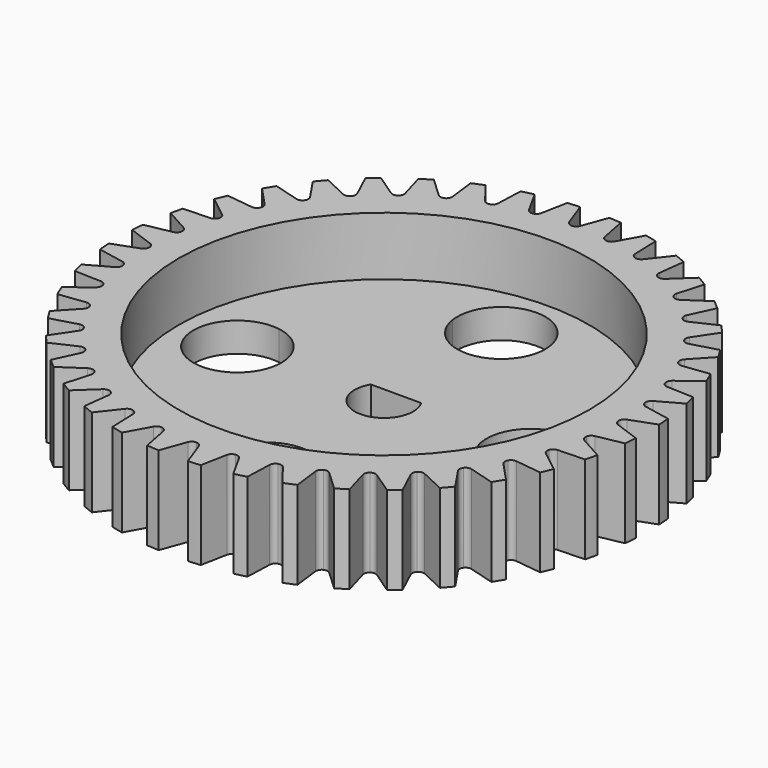
from build123d import *

# Parameters (mm, degrees)
F0_R            = 35
F0_R_2          = 10
F1_DEPTH        = 5
F2_DEPTH        = 15
F3_R            = 2
F4_DEPTH        = 32.4449635407
F0_R_3          = 45
F0_R_4          = 40
F5_DEPTH        = 5
F6_DEPTH        = 10
F8_DEPTH        = 25.0010001
F8_COPIES_COUNT = 40


# Not quite as in the source:
# - a feature of the source that left no trace in its solid (it failed there, or was rolled back) is left out
# - a pattern or mirror of a feature is missing from the dataset's text; its kind, count and spacing are read off the source's solid


with BuildPart() as f1:
    # F0 (on Top) → F1 (new body)
    with BuildSketch(Plane.XY):
        Circle(F0_R)
        with BuildLine():
            ThreePointArc((7.415144975, 23.875), (17.6776695297, 17.6776695297), (23.875, 7.415144975))
            ThreePointArc((23.875, 7.415144975), (29.8894018039, 5.687156583), (32.5, 0))
            ThreePointArc((32.5, 0), (29.8894018039, -5.687156583), (23.875, -7.415144975))
            ThreePointArc((23.875, -7.415144975), (17.6776695297, -17.6776695297), (7.415144975, -23.875))
            ThreePointArc((7.415144975, -23.875), (7.478756157, -24.4359021859), (7.5, -25))
            ThreePointArc((7.5, -25), (-0.5640978141, -32.478756157), (-7.415144975, -23.875))
            ThreePointArc((-7.415144975, -23.875), (-17.6776695297, -17.6776695297), (-23.875, -7.415144975))
            ThreePointArc((-23.875, -7.415144975), (-32.5, 0), (-23.875, 7.415144975))
            ThreePointArc((-23.875, 7.415144975), (-17.6776695297, 17.6776695297), (-7.415144975, 23.875))
            ThreePointArc((-7.415144975, 23.875), (-0.5640978141, 32.478756157), (7.5, 25))
            ThreePointArc((7.5, 25), (7.478756157, 24.4359021859), (7.415144975, 23.875))
        make_face(mode=Mode.SUBTRACT)
        with BuildLine():
            ThreePointArc((23.875, -7.415144975), (17.5, 0), (23.875, 7.415144975))
            ThreePointArc((23.875, 7.415144975), (17.6776695297, 17.6776695297), (7.415144975, 23.875))
            ThreePointArc((7.415144975, 23.875), (0, 17.5), (-7.415144975, 23.875))
            ThreePointArc((-7.415144975, 23.875), (-17.6776695297, 17.6776695297), (-23.875, 7.415144975))
            ThreePointArc((-23.875, 7.415144975), (-19.312843417, 4.8894018039), (-17.5, 0))
            ThreePointArc((-17.5, 0), (-19.312843417, -4.8894018039), (-23.875, -7.415144975))
            ThreePointArc((-23.875, -7.415144975), (-17.6776695297, -17.6776695297), (-7.415144975, -23.875))
            ThreePointArc((-7.415144975, -23.875), (0, -17.5), (7.415144975, -23.875))
            ThreePointArc((7.415144975, -23.875), (17.6776695297, -17.6776695297), (23.875, -7.415144975))
        make_face()
        Circle(F0_R_2, mode=Mode.SUBTRACT)
    extrude(amount=-F1_DEPTH)

    # F0 (on Top) → F2 (join)
    with BuildSketch(Plane.XY):
        Circle(F0_R_2)
        with BuildLine():
            ThreePointArc((5, 0), (-1.3254364946, -4.8211220788), (-4.2972872395, 2.5560364593))
            ThreePointArc((-4.2972872395, 2.5560364593), (0, 5), (4.2972872395, 2.5560364593))
            ThreePointArc((4.2972872395, 2.5560364593), (4.8211220788, 1.3254364946), (5, 0))
        make_face(mode=Mode.SUBTRACT)
        with BuildLine():
            ThreePointArc((4.2972872395, 2.5560364593), (0, 5), (-4.2972872395, 2.5560364593))
            Line((-4.2972872395, 2.5560364593), (4.2972872395, 2.5560364593))
        make_face()
    extrude(amount=-F2_DEPTH)

    # F3 (on face) → F4 (cut, through all)
    with BuildSketch(Plane.XZ.offset(-2.5560364593)):
        with Locations((0, -10)):
            Circle(F3_R)
    extrude(amount=-F4_DEPTH, mode=Mode.SUBTRACT)

    # F0 (on Top) → F5 (join)
    with BuildSketch(Plane.XY):
        Circle(F0_R_3)
        Circle(F0_R_4, mode=Mode.SUBTRACT)
        Circle(F0_R_4)
        Circle(F0_R, mode=Mode.SUBTRACT)
    extrude(amount=-F5_DEPTH)

    # F0 (on Top) → F6 (join)
    with BuildSketch(Plane.XY):
        Circle(F0_R_3)
        Circle(F0_R_4, mode=Mode.SUBTRACT)
        Circle(F0_R_4)
        Circle(F0_R, mode=Mode.SUBTRACT)
    extrude(amount=F6_DEPTH)

    # F7 (on face) → F8 (cut, through all)
    with BuildSketch(Plane.XY.offset(10)):
        with BuildLine():
            Line((0.9396926208, 40.6579798567), (2.4948673053, 44.9307871857))
            ThreePointArc((2.4948673053, 44.9307871857), (0, 45), (-2.4948673053, 44.9307871857))
            Line((-2.4948673053, 44.9307871857), (-0.9396926208, 40.6579798567))
            ThreePointArc((-0.9396926208, 40.6579798567), (-0.5735764364, 40.1808479557), (0, 40))
            ThreePointArc((0, 40), (0.5735764364, 40.1808479557), (0.9396926208, 40.6579798567))
        make_face()
    f8 = extrude(amount=-F8_DEPTH, mode=Mode.SUBTRACT)

    # F8_copies: F8 ×40 about axis
    f8_copies_axis = Axis((0, 0, 0), (0, 0, 1))
    for i in range(1, F8_COPIES_COUNT):
        add(f8.rotate(f8_copies_axis, i * 360 / F8_COPIES_COUNT), mode=Mode.SUBTRACT)


solid = f1.part
